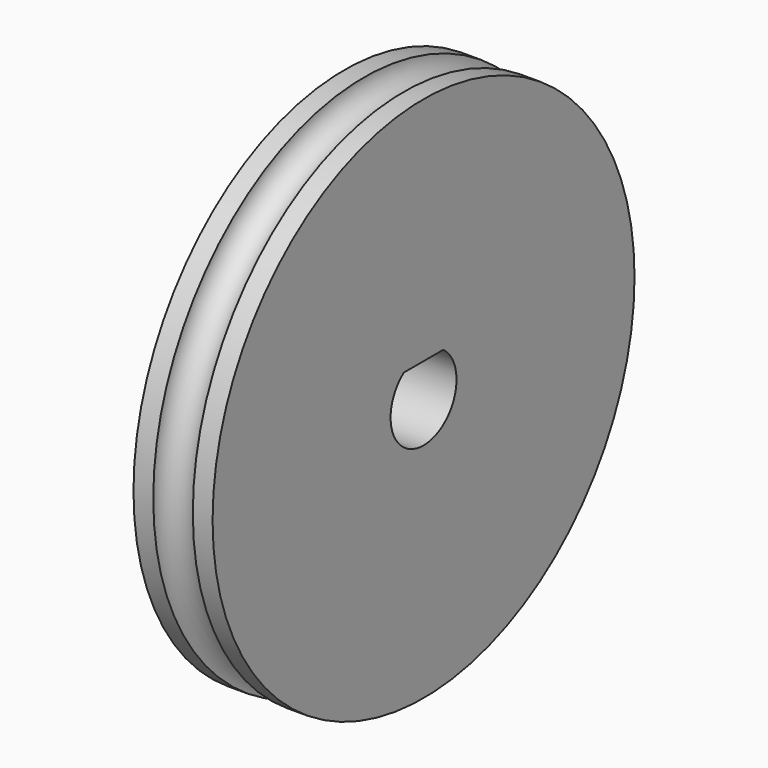
from build123d import *

# Parameters (mm, degrees)
F3_R      = 5
F4_DEPTH  = 5
F7_DEPTH  = 11
F9_R      = 2.45
F10_DEPTH = 5
F12_R     = 0.95
F13_DEPTH = 5


# Not quite as in the source:
# - ends of sketch curves that miss each other by under 0.0002 mm in the source are joined


with BuildPart() as f1:
    # F0 (on Top) → F1 (revolve)
    with BuildSketch(Plane.XY):
        with BuildLine():
            Line((-4.5, 0), (1.5, 0))
            Line((1.5, 0), (1.5, 20))
            Line((1.5, 20), (0, 20))
            ThreePointArc((0, 20), (-1.5, 18.4999958554), (-3.0000041446, 20))
            Line((-3.0000041446, 20), (-4.5, 20))
            Line((-4.5, 20), (-4.5, 0))
        make_face()
    revolve(axis=Axis((-1.5, 0, 0), (1, 0, 0)))

    # F3 (on offset) → F4 (join)
    with BuildSketch(Plane(origin=(-4.5, 0, 0), x_dir=(0, -1, 0), z_dir=(-1, 0, 0))):
        Circle(F3_R)
    extrude(amount=F4_DEPTH)

    # F6 (on offset) → F7 (cut, through all)
    with BuildSketch(Plane(origin=(-9.5, 0, 0), x_dir=(0, -1, 0), z_dir=(-1, 0, 0))):
        with BuildLine():
            Line((1.875, 2.5), (-1.875, 2.5))
            ThreePointArc((-1.875, 2.5), (0, -3.125), (1.875, 2.5))
        make_face()
    extrude(amount=-F7_DEPTH, mode=Mode.SUBTRACT)

    # F9 (on offset) → F10 (join)
    with BuildSketch(Plane(origin=(0, 0, 2.5), x_dir=(1, 0, 0), z_dir=(0, 0, -1))):
        with Locations((-7, 0)):
            Circle(F9_R)
    extrude(amount=-F10_DEPTH)

    # F12 (on offset) → F13 (cut, through all)
    with BuildSketch(Plane.XY.offset(7.5)):
        with Locations((-7, 0)):
            Circle(F12_R)
    extrude(amount=-F13_DEPTH, mode=Mode.SUBTRACT)


solid = f1.part
